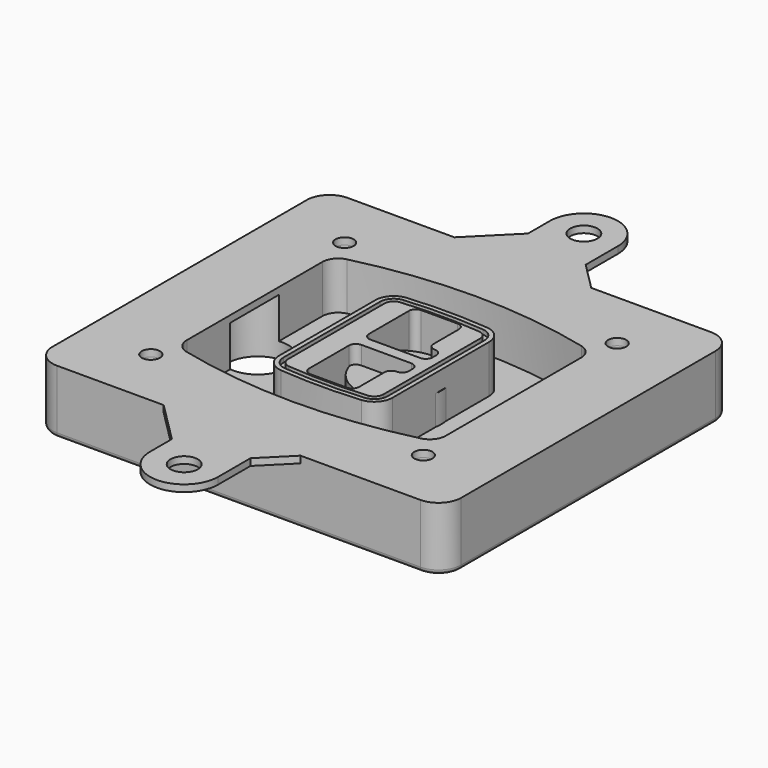
from build123d import *

# Parameters (mm, degrees)
F0_R      = 4
F1_DEPTH  = 25
F2_DEPTH  = 3
F3_DEPTH  = 18
F5_DEPTH  = 21
F6_DEPTH  = 2
F8_DEPTH  = 20
F9_DEPTH  = 16
F10_DEPTH = 25
F7_R      = 6
F7_R_2    = 4
F11_DEPTH = 6
F13_DEPTH = 9
F15_R     = 2
F16_R     = 4
F16_R_2   = 6
F17_DEPTH = 3


# Not quite as in the source:
# - a feature of the source that left no trace in its solid (it failed there, or was rolled back) is left out
# - a feature names something its author has since deleted; it is built from what else it names


with BuildPart() as f1:
    # F0 (on Top) → F1 (new body)
    with BuildSketch(Plane.XY):
        with BuildLine():
            ThreePointArc((-90, -70), (-87.0710678119, -77.0710678119), (-80, -80))
            Line((-80, -80), (80, -80))
            ThreePointArc((80, -80), (87.0710678119, -77.0710678119), (90, -70))
            Line((90, -70), (90, 70))
            ThreePointArc((90, 70), (87.0710678119, 77.0710678119), (80, 80))
            Line((80, 80), (-80, 80))
            ThreePointArc((-80, 80), (-87.0710678119, 77.0710678119), (-90, 70))
            Line((-90, 70), (-90, -70))
        make_face()
        with Locations((-60, -53.3333333333)):
            Circle(F0_R, mode=Mode.SUBTRACT)
        with Locations((60, -53.3333333333)):
            Circle(F0_R, mode=Mode.SUBTRACT)
        with Locations((-60, 53.3333333333)):
            Circle(F0_R, mode=Mode.SUBTRACT)
        with BuildLine():
            ThreePointArc((-64, 37.2990447398), (-61.0143011354, 45.9411029726), (-53.3306899286, 50.8970778549))
            ThreePointArc((-53.3306899286, 50.8970778549), (0, 57.3333333333), (53.3306899286, 50.8970778549))
            ThreePointArc((53.3306899286, 50.8970778549), (61.0143011354, 45.9411029726), (64, 37.2990447398))
            Line((64, 37.2990447398), (64, -37.2990447398))
            ThreePointArc((64, -37.2990447398), (61.0143011354, -45.9411029726), (53.3306899286, -50.8970778549))
            ThreePointArc((53.3306899286, -50.8970778549), (0, -57.3333333333), (-53.3306899286, -50.8970778549))
            ThreePointArc((-53.3306899286, -50.8970778549), (-61.0143011354, -45.9411029726), (-64, -37.2990447398))
            Line((-64, -37.2990447398), (-64, 37.2990447398))
        make_face(mode=Mode.SUBTRACT)
        with Locations((60, 53.3333333333)):
            Circle(F0_R, mode=Mode.SUBTRACT)
        with BuildLine():
            ThreePointArc((53.3306899286, 50.8970778549), (0, 57.3333333333), (-53.3306899286, 50.8970778549))
            ThreePointArc((-53.3306899286, 50.8970778549), (-61.0143011354, 45.9411029726), (-64, 37.2990447398))
            Line((-64, 37.2990447398), (-64, -37.2990447398))
            ThreePointArc((-64, -37.2990447398), (-61.0143011354, -45.9411029726), (-53.3306899286, -50.8970778549))
            ThreePointArc((-53.3306899286, -50.8970778549), (0, -57.3333333333), (53.3306899286, -50.8970778549))
            ThreePointArc((53.3306899286, -50.8970778549), (61.0143011354, -45.9411029726), (64, -37.2990447398))
            Line((64, -37.2990447398), (64, 37.2990447398))
            ThreePointArc((64, 37.2990447398), (61.0143011354, 45.9411029726), (53.3306899286, 50.8970778549))
        make_face()
        with BuildLine():
            Line((-60, -37.2990447398), (-60, 37.2990447398))
            ThreePointArc((-60, 37.2990447398), (-57.8673579538, 43.4719434775), (-52.3790642347, 47.0119255363))
            ThreePointArc((-52.3790642347, 47.0119255363), (0, 53.3333333333), (52.3790642347, 47.0119255363))
            ThreePointArc((52.3790642347, 47.0119255363), (57.8673579538, 43.4719434775), (60, 37.2990447398))
            Line((60, 37.2990447398), (60, -37.2990447398))
            ThreePointArc((60, -37.2990447398), (57.8673579538, -43.4719434775), (52.3790642347, -47.0119255363))
            ThreePointArc((52.3790642347, -47.0119255363), (0, -53.3333333333), (-52.3790642347, -47.0119255363))
            ThreePointArc((-52.3790642347, -47.0119255363), (-57.8673579538, -43.4719434775), (-60, -37.2990447398))
        make_face(mode=Mode.SUBTRACT)
        with BuildLine():
            ThreePointArc((-52.3790642347, 47.0119255363), (-57.8673579538, 43.4719434775), (-60, 37.2990447398))
            Line((-60, 37.2990447398), (-60, -37.2990447398))
            ThreePointArc((-60, -37.2990447398), (-57.8673579538, -43.4719434775), (-52.3790642347, -47.0119255363))
            ThreePointArc((-52.3790642347, -47.0119255363), (0, -53.3333333333), (52.3790642347, -47.0119255363))
            ThreePointArc((52.3790642347, -47.0119255363), (57.8673579538, -43.4719434775), (60, -37.2990447398))
            Line((60, -37.2990447398), (60, 37.2990447398))
            ThreePointArc((60, 37.2990447398), (57.8673579538, 43.4719434775), (52.3790642347, 47.0119255363))
            ThreePointArc((52.3790642347, 47.0119255363), (0, 53.3333333333), (-52.3790642347, 47.0119255363))
        make_face()
        with BuildLine():
            ThreePointArc((51.6653449643, 44.0980612973), (55.5071505677, 41.6200738562), (57, 37.2990447398))
            Line((57, 37.2990447398), (57, -37.2990447398))
            ThreePointArc((57, -37.2990447398), (55.5071505677, -41.6200738562), (51.6653449643, -44.0980612973))
            ThreePointArc((51.6653449643, -44.0980612973), (0, -50.3333333333), (-51.6653449643, -44.0980612973))
            ThreePointArc((-51.6653449643, -44.0980612973), (-55.5071505677, -41.6200738562), (-57, -37.2990447398))
            Line((-57, -37.2990447398), (-57, 37.2990447398))
            ThreePointArc((-57, 37.2990447398), (-55.5071505677, 41.6200738562), (-51.6653449643, 44.0980612973))
            ThreePointArc((-51.6653449643, 44.0980612973), (0, 50.3333333333), (51.6653449643, 44.0980612973))
        make_face(mode=Mode.SUBTRACT)
        with BuildLine():
            Line((57, -37.2990447398), (57, 37.2990447398))
            ThreePointArc((57, 37.2990447398), (55.5071505677, 41.6200738562), (51.6653449643, 44.0980612973))
            ThreePointArc((51.6653449643, 44.0980612973), (0, 50.3333333333), (-51.6653449643, 44.0980612973))
            ThreePointArc((-51.6653449643, 44.0980612973), (-55.5071505677, 41.6200738562), (-57, 37.2990447398))
            Line((-57, 37.2990447398), (-57, -37.2990447398))
            ThreePointArc((-57, -37.2990447398), (-55.5071505677, -41.6200738562), (-51.6653449643, -44.0980612973))
            ThreePointArc((-51.6653449643, -44.0980612973), (0, -50.3333333333), (51.6653449643, -44.0980612973))
            ThreePointArc((51.6653449643, -44.0980612973), (55.5071505677, -41.6200738562), (57, -37.2990447398))
        make_face()
    extrude(amount=-F1_DEPTH)

    # F0 (on Top) → F2 (join)
    with BuildSketch(Plane.XY):
        with BuildLine():
            ThreePointArc((-52.3790642347, 47.0119255363), (-57.8673579538, 43.4719434775), (-60, 37.2990447398))
            Line((-60, 37.2990447398), (-60, -37.2990447398))
            ThreePointArc((-60, -37.2990447398), (-57.8673579538, -43.4719434775), (-52.3790642347, -47.0119255363))
            ThreePointArc((-52.3790642347, -47.0119255363), (0, -53.3333333333), (52.3790642347, -47.0119255363))
            ThreePointArc((52.3790642347, -47.0119255363), (57.8673579538, -43.4719434775), (60, -37.2990447398))
            Line((60, -37.2990447398), (60, 37.2990447398))
            ThreePointArc((60, 37.2990447398), (57.8673579538, 43.4719434775), (52.3790642347, 47.0119255363))
            ThreePointArc((52.3790642347, 47.0119255363), (0, 53.3333333333), (-52.3790642347, 47.0119255363))
        make_face()
        with BuildLine():
            ThreePointArc((51.6653449643, 44.0980612973), (55.5071505677, 41.6200738562), (57, 37.2990447398))
            Line((57, 37.2990447398), (57, -37.2990447398))
            ThreePointArc((57, -37.2990447398), (55.5071505677, -41.6200738562), (51.6653449643, -44.0980612973))
            ThreePointArc((51.6653449643, -44.0980612973), (0, -50.3333333333), (-51.6653449643, -44.0980612973))
            ThreePointArc((-51.6653449643, -44.0980612973), (-55.5071505677, -41.6200738562), (-57, -37.2990447398))
            Line((-57, -37.2990447398), (-57, 37.2990447398))
            ThreePointArc((-57, 37.2990447398), (-55.5071505677, 41.6200738562), (-51.6653449643, 44.0980612973))
            ThreePointArc((-51.6653449643, 44.0980612973), (0, 50.3333333333), (51.6653449643, 44.0980612973))
        make_face(mode=Mode.SUBTRACT)
    extrude(amount=F2_DEPTH)

    # F0 (on Top) → F3 (cut)
    with BuildSketch(Plane.XY):
        with BuildLine():
            Line((57, -37.2990447398), (57, 37.2990447398))
            ThreePointArc((57, 37.2990447398), (55.5071505677, 41.6200738562), (51.6653449643, 44.0980612973))
            ThreePointArc((51.6653449643, 44.0980612973), (0, 50.3333333333), (-51.6653449643, 44.0980612973))
            ThreePointArc((-51.6653449643, 44.0980612973), (-55.5071505677, 41.6200738562), (-57, 37.2990447398))
            Line((-57, 37.2990447398), (-57, -37.2990447398))
            ThreePointArc((-57, -37.2990447398), (-55.5071505677, -41.6200738562), (-51.6653449643, -44.0980612973))
            ThreePointArc((-51.6653449643, -44.0980612973), (0, -50.3333333333), (51.6653449643, -44.0980612973))
            ThreePointArc((51.6653449643, -44.0980612973), (55.5071505677, -41.6200738562), (57, -37.2990447398))
        make_face()
    extrude(amount=-F3_DEPTH, mode=Mode.SUBTRACT)

    # F4 (on face) → F5 (join, through all)
    with BuildSketch(Plane.XY.offset(3)):
        with BuildLine():
            ThreePointArc((-25, -26.587695628), (-22.8992979869, -31.9912392117), (-17.7004291845, -34.5569740744))
            ThreePointArc((-17.7004291845, -34.5569740744), (0, -35.3333333333), (17.7004291845, -34.5569740744))
            ThreePointArc((17.7004291845, -34.5569740744), (22.8992979869, -31.9912392117), (25, -26.587695628))
            Line((25, -26.587695628), (25, 26.587695628))
            ThreePointArc((25, 26.587695628), (22.8992979869, 31.9912392117), (17.7004291845, 34.5569740744))
            ThreePointArc((17.7004291845, 34.5569740744), (0, 35.3333333333), (-17.7004291845, 34.5569740744))
            ThreePointArc((-17.7004291845, 34.5569740744), (-22.8992979869, 31.9912392117), (-25, 26.587695628))
            Line((-25, 26.587695628), (-25, -26.587695628))
        make_face()
        with BuildLine():
            ThreePointArc((17.5253218884, 32.5646544628), (21.4244734902, 30.6403533158), (23, 26.587695628))
            Line((23, 26.587695628), (23, -26.587695628))
            ThreePointArc((23, -26.587695628), (21.4244734902, -30.6403533158), (17.5253218884, -32.5646544628))
            ThreePointArc((17.5253218884, -32.5646544628), (0, -33.3333333333), (-17.5253218884, -32.5646544628))
            ThreePointArc((-17.5253218884, -32.5646544628), (-21.4244734902, -30.6403533158), (-23, -26.587695628))
            Line((-23, -26.587695628), (-23, 26.587695628))
            ThreePointArc((-23, 26.587695628), (-21.4244734902, 30.6403533158), (-17.5253218884, 32.5646544628))
            ThreePointArc((-17.5253218884, 32.5646544628), (0, 33.3333333333), (17.5253218884, 32.5646544628))
        make_face(mode=Mode.SUBTRACT)
        with BuildLine():
            Line((23, -26.587695628), (23, 26.587695628))
            ThreePointArc((23, 26.587695628), (21.4244734902, 30.6403533158), (17.5253218884, 32.5646544628))
            ThreePointArc((17.5253218884, 32.5646544628), (0, 33.3333333333), (-17.5253218884, 32.5646544628))
            ThreePointArc((-17.5253218884, 32.5646544628), (-21.4244734902, 30.6403533158), (-23, 26.587695628))
            Line((-23, 26.587695628), (-23, -26.587695628))
            ThreePointArc((-23, -26.587695628), (-21.4244734902, -30.6403533158), (-17.5253218884, -32.5646544628))
            ThreePointArc((-17.5253218884, -32.5646544628), (0, -33.3333333333), (17.5253218884, -32.5646544628))
            ThreePointArc((17.5253218884, -32.5646544628), (21.4244734902, -30.6403533158), (23, -26.587695628))
        make_face()
        with BuildLine():
            ThreePointArc((17.3502145923, 30.5723348512), (19.9496489934, 29.2894674198), (21, 26.587695628))
            Line((21, 26.587695628), (21, -26.587695628))
            ThreePointArc((21, -26.587695628), (19.9496489934, -29.2894674198), (17.3502145923, -30.5723348512))
            ThreePointArc((17.3502145923, -30.5723348512), (0, -31.3333333333), (-17.3502145923, -30.5723348512))
            ThreePointArc((-17.3502145923, -30.5723348512), (-19.9496489934, -29.2894674198), (-21, -26.587695628))
            Line((-21, -26.587695628), (-21, 26.587695628))
            ThreePointArc((-21, 26.587695628), (-19.9496489934, 29.2894674198), (-17.3502145923, 30.5723348512))
            ThreePointArc((-17.3502145923, 30.5723348512), (0, 31.3333333333), (17.3502145923, 30.5723348512))
        make_face(mode=Mode.SUBTRACT)
        with BuildLine():
            Line((21, -26.587695628), (21, 26.587695628))
            ThreePointArc((21, 26.587695628), (19.9496489934, 29.2894674198), (17.3502145923, 30.5723348512))
            ThreePointArc((17.3502145923, 30.5723348512), (0, 31.3333333333), (-17.3502145923, 30.5723348512))
            ThreePointArc((-17.3502145923, 30.5723348512), (-19.9496489934, 29.2894674198), (-21, 26.587695628))
            Line((-21, 26.587695628), (-21, -26.587695628))
            ThreePointArc((-21, -26.587695628), (-19.9496489934, -29.2894674198), (-17.3502145923, -30.5723348512))
            ThreePointArc((-17.3502145923, -30.5723348512), (0, -31.3333333333), (17.3502145923, -30.5723348512))
            ThreePointArc((17.3502145923, -30.5723348512), (19.9496489934, -29.2894674198), (21, -26.587695628))
        make_face()
        with BuildLine():
            Line((-8, -2.5), (14, -2.5))
            ThreePointArc((14, -2.5), (16.1213203436, -3.3786796564), (17, -5.5))
            Line((17, -5.5), (17, -7.5))
            ThreePointArc((17, -7.5), (16.1213203436, -9.6213203436), (14, -10.5))
            ThreePointArc((14, -10.5), (11.8786796564, -11.3786796564), (11, -13.5))
            Line((11, -13.5), (11, -27.5))
            ThreePointArc((11, -27.5), (10.1213203436, -29.6213203436), (8, -30.5))
            Line((8, -30.5), (-8, -30.5))
            ThreePointArc((-8, -30.5), (-10.1213203436, -29.6213203436), (-11, -27.5))
            Line((-11, -27.5), (-11, -5.5))
            ThreePointArc((-11, -5.5), (-10.1213203436, -3.3786796564), (-8, -2.5))
        make_face(mode=Mode.SUBTRACT)
        with BuildLine():
            ThreePointArc((-8, 2.5), (-10.1213203436, 3.3786796564), (-11, 5.5))
            Line((-11, 5.5), (-11, 27.5))
            ThreePointArc((-11, 27.5), (-10.1213203436, 29.6213203436), (-8, 30.5))
            Line((-8, 30.5), (8, 30.5))
            ThreePointArc((8, 30.5), (10.1213203436, 29.6213203436), (11, 27.5))
            Line((11, 27.5), (11, 13.5))
            ThreePointArc((11, 13.5), (11.8786796564, 11.3786796564), (14, 10.5))
            ThreePointArc((14, 10.5), (16.1213203436, 9.6213203436), (17, 7.5))
            Line((17, 7.5), (17, 5.5))
            ThreePointArc((17, 5.5), (16.1213203436, 3.3786796564), (14, 2.5))
            Line((14, 2.5), (-8, 2.5))
        make_face(mode=Mode.SUBTRACT)
    extrude(amount=-F5_DEPTH)

    # F4 (on face) → F6 (cut)
    with BuildSketch(Plane.XY.offset(3)):
        with BuildLine():
            Line((23, -26.587695628), (23, 26.587695628))
            ThreePointArc((23, 26.587695628), (21.4244734902, 30.6403533158), (17.5253218884, 32.5646544628))
            ThreePointArc((17.5253218884, 32.5646544628), (0, 33.3333333333), (-17.5253218884, 32.5646544628))
            ThreePointArc((-17.5253218884, 32.5646544628), (-21.4244734902, 30.6403533158), (-23, 26.587695628))
            Line((-23, 26.587695628), (-23, -26.587695628))
            ThreePointArc((-23, -26.587695628), (-21.4244734902, -30.6403533158), (-17.5253218884, -32.5646544628))
            ThreePointArc((-17.5253218884, -32.5646544628), (0, -33.3333333333), (17.5253218884, -32.5646544628))
            ThreePointArc((17.5253218884, -32.5646544628), (21.4244734902, -30.6403533158), (23, -26.587695628))
        make_face()
        with BuildLine():
            ThreePointArc((17.3502145923, 30.5723348512), (19.9496489934, 29.2894674198), (21, 26.587695628))
            Line((21, 26.587695628), (21, -26.587695628))
            ThreePointArc((21, -26.587695628), (19.9496489934, -29.2894674198), (17.3502145923, -30.5723348512))
            ThreePointArc((17.3502145923, -30.5723348512), (0, -31.3333333333), (-17.3502145923, -30.5723348512))
            ThreePointArc((-17.3502145923, -30.5723348512), (-19.9496489934, -29.2894674198), (-21, -26.587695628))
            Line((-21, -26.587695628), (-21, 26.587695628))
            ThreePointArc((-21, 26.587695628), (-19.9496489934, 29.2894674198), (-17.3502145923, 30.5723348512))
            ThreePointArc((-17.3502145923, 30.5723348512), (0, 31.3333333333), (17.3502145923, 30.5723348512))
        make_face(mode=Mode.SUBTRACT)
    extrude(amount=-F6_DEPTH, mode=Mode.SUBTRACT)

    # F7 (on face) → F8 (join)
    with BuildSketch(Plane(origin=(0, 0, -25), x_dir=(1, 0, 0), z_dir=(0, 0, -1))):
        with BuildLine():
            ThreePointArc((-6.71157564, 0), (6.7567035675, 13.4682792075), (20.224982775, 0))
            Line((20.224982775, 0), (25.224982775, 0))
            ThreePointArc((25.224982775, 0), (6.7567035675, 18.4682792075), (-11.71157564, 0))
            Line((-11.71157564, 0), (-6.71157564, 0))
        make_face()
        with BuildLine():
            Line((-6.71157564, 0), (20.224982775, 0))
            ThreePointArc((20.224982775, 0), (6.7567035675, 13.4682792075), (-6.71157564, 0))
        make_face()
        with BuildLine():
            ThreePointArc((-6.71157564, 0), (6.7567035675, -13.4682792075), (20.224982775, 0))
            Line((20.224982775, 0), (-6.71157564, 0))
        make_face()
        with BuildLine():
            Line((25.224982775, 0), (20.224982775, 0))
            ThreePointArc((20.224982775, 0), (6.7567035675, -13.4682792075), (-6.71157564, 0))
            Line((-6.71157564, 0), (-11.71157564, 0))
            ThreePointArc((-11.71157564, 0), (6.7567035675, -18.4682792075), (25.224982775, 0))
        make_face()
    extrude(amount=-F8_DEPTH)

    # F7 (on face) → F9 (cut)
    with BuildSketch(Plane(origin=(0, 0, -25), x_dir=(1, 0, 0), z_dir=(0, 0, -1))):
        with BuildLine():
            Line((-6.71157564, 0), (20.224982775, 0))
            ThreePointArc((20.224982775, 0), (6.7567035675, 13.4682792075), (-6.71157564, 0))
        make_face()
        with BuildLine():
            ThreePointArc((-6.71157564, 0), (6.7567035675, -13.4682792075), (20.224982775, 0))
            Line((20.224982775, 0), (-6.71157564, 0))
        make_face()
    extrude(amount=-F9_DEPTH, mode=Mode.SUBTRACT)

    # F7 (on face) → F10 (cut)
    with BuildSketch(Plane(origin=(0, 0, -25), x_dir=(1, 0, 0), z_dir=(0, 0, -1))):
        with BuildLine():
            Line((-69.0318229325, 0), (-42.0952645175, 0))
            ThreePointArc((-42.0952645175, 0), (-55.563543725, 13.4682792075), (-69.0318229325, 0))
        make_face()
        with BuildLine():
            ThreePointArc((-69.0318229325, 0), (-55.563543725, -13.4682792075), (-42.0952645175, 0))
            Line((-42.0952645175, 0), (-69.0318229325, 0))
        make_face()
    extrude(amount=-F10_DEPTH, mode=Mode.SUBTRACT)

    # F7 (on face) → F11 (cut)
    with BuildSketch(Plane(origin=(0, 0, -25), x_dir=(1, 0, 0), z_dir=(0, 0, -1))):
        with Locations((60, -53.3333333333)):
            Circle(F7_R)
        with Locations((60, -53.3333333333)):
            Circle(F7_R_2, mode=Mode.SUBTRACT)
        with Locations((-60, -53.3333333333)):
            Circle(F7_R)
        with Locations((-60, -53.3333333333)):
            Circle(F7_R_2, mode=Mode.SUBTRACT)
        with Locations((-60, 53.3333333333)):
            Circle(F7_R)
        with Locations((-60, 53.3333333333)):
            Circle(F7_R_2, mode=Mode.SUBTRACT)
        with Locations((60, 53.3333333333)):
            Circle(F7_R)
        with Locations((60, 53.3333333333)):
            Circle(F7_R_2, mode=Mode.SUBTRACT)
    extrude(amount=-F11_DEPTH, mode=Mode.SUBTRACT)

    # F12 (on face) → F13 (cut, through all)
    with BuildSketch(Plane(origin=(0, 0, -9), x_dir=(1, 0, 0), z_dir=(0, 0, -1))):
        with BuildLine():
            ThreePointArc((20.224982775, 0), (20.1663399806, 1.2554664788), (19.9909222755, 2.5))
            Line((19.9909222755, 2.5), (14, 2.5))
            ThreePointArc((14, 2.5), (16.1213203436, 3.3786796564), (17, 5.5))
            Line((17, 5.5), (17, 7.5))
            ThreePointArc((17, 7.5), (16.1213203436, 9.6213203436), (14, 10.5))
            ThreePointArc((14, 10.5), (12.1627255951, 11.1284134507), (11.0951631559, 12.750384826))
            ThreePointArc((11.0951631559, 12.750384826), (11.0476113807, 12.7664660322), (11, 12.7823698976))
            Line((11, 12.7823698976), (11, -12.7823698976))
            ThreePointArc((11, -12.7823698976), (11.0476113807, -12.7664660322), (11.0951631559, -12.750384826))
            ThreePointArc((11.0951631559, -12.750384826), (12.1627255951, -11.1284134507), (14, -10.5))
            ThreePointArc((14, -10.5), (16.1213203436, -9.6213203436), (17, -7.5))
            Line((17, -7.5), (17, -5.5))
            ThreePointArc((17, -5.5), (16.1213203436, -3.3786796564), (14, -2.5))
            Line((14, -2.5), (19.9909222755, -2.5))
            ThreePointArc((19.9909222755, -2.5), (20.1663399806, -1.2554664788), (20.224982775, 0))
        make_face()
    extrude(amount=F13_DEPTH, mode=Mode.SUBTRACT)

    # F15
    f15_edges = [f1.edges().sort_by_distance(p)[0] for p in [
        (0, -80, -25),
        (-87.071068, -77.071068, -25),
        (-90, 0, -25),
        (-87.071068, 77.071068, -25),
        (87.071068, -77.071068, -25),
        (0, 80, -25),
        (90, 0, -25),
        (87.071068, 77.071068, -25),
    ]]
    fillet(f15_edges, radius=F15_R)

    # F16 (on Top) → F17 (join, through all)
    with BuildSketch(Plane.XY):
        with BuildLine():
            ThreePointArc((80, -80), (87.0710678119, -77.0710678119), (90, -70))
            Line((90, -70), (90, 70))
            ThreePointArc((90, 70), (87.0710678119, 77.0710678119), (80, 80))
            Line((80, 80), (27.25, 80))
            Line((27.25, 80), (-33, 80))
            Line((-33, 80), (-80, 80))
            ThreePointArc((-80, 80), (-87.0710678119, 77.0710678119), (-90, 70))
            Line((-90, 70), (-90, -70))
            ThreePointArc((-90, -70), (-87.0710678119, -77.0710678119), (-80, -80))
            Line((-80, -80), (-33, -80))
            Line((-33, -80), (27.25, -80))
            Line((27.25, -80), (80, -80))
        make_face()
        with Locations((-60, -53.3333333333)):
            Circle(F16_R, mode=Mode.SUBTRACT)
        with Locations((60, -53.3333333333)):
            Circle(F16_R, mode=Mode.SUBTRACT)
        with Locations((-60, 53.3333333333)):
            Circle(F16_R, mode=Mode.SUBTRACT)
        with BuildLine():
            ThreePointArc((52.3790642347, -47.0119255363), (0, -53.3333333333), (-52.3790642347, -47.0119255363))
            ThreePointArc((-52.3790642347, -47.0119255363), (-57.8673579538, -43.4719434775), (-60, -37.2990447398))
            Line((-60, -37.2990447398), (-60, 37.2990447398))
            ThreePointArc((-60, 37.2990447398), (-57.8673579538, 43.4719434775), (-52.3790642347, 47.0119255363))
            ThreePointArc((-52.3790642347, 47.0119255363), (0, 53.3333333333), (52.3790642347, 47.0119255363))
            ThreePointArc((52.3790642347, 47.0119255363), (57.8673579538, 43.4719434775), (60, 37.2990447398))
            Line((60, 37.2990447398), (60, -37.2990447398))
            ThreePointArc((60, -37.2990447398), (57.8673579538, -43.4719434775), (52.3790642347, -47.0119255363))
        make_face(mode=Mode.SUBTRACT)
        with Locations((60, 53.3333333333)):
            Circle(F16_R, mode=Mode.SUBTRACT)
        with BuildLine():
            Line((15, -92.25), (27.25, -80))
            Line((27.25, -80), (-33, -80))
            Line((-33, -80), (-15, -98))
            Line((-15, -98), (-15, -110))
            ThreePointArc((-15, -110), (0, -125), (15, -110))
            Line((15, -110), (15, -92.25))
        make_face()
        with Locations((0, -110)):
            Circle(F16_R_2, mode=Mode.SUBTRACT)
        with BuildLine():
            Line((-33, 80), (27.25, 80))
            Line((27.25, 80), (15, 92.25))
            Line((15, 92.25), (15, 110))
            ThreePointArc((15, 110), (0, 125), (-15, 110))
            Line((-15, 110), (-15, 98))
            Line((-15, 98), (-33, 80))
        make_face()
        with Locations((0, 110)):
            Circle(F16_R_2, mode=Mode.SUBTRACT)
    extrude(amount=F17_DEPTH)


solid = f1.part
